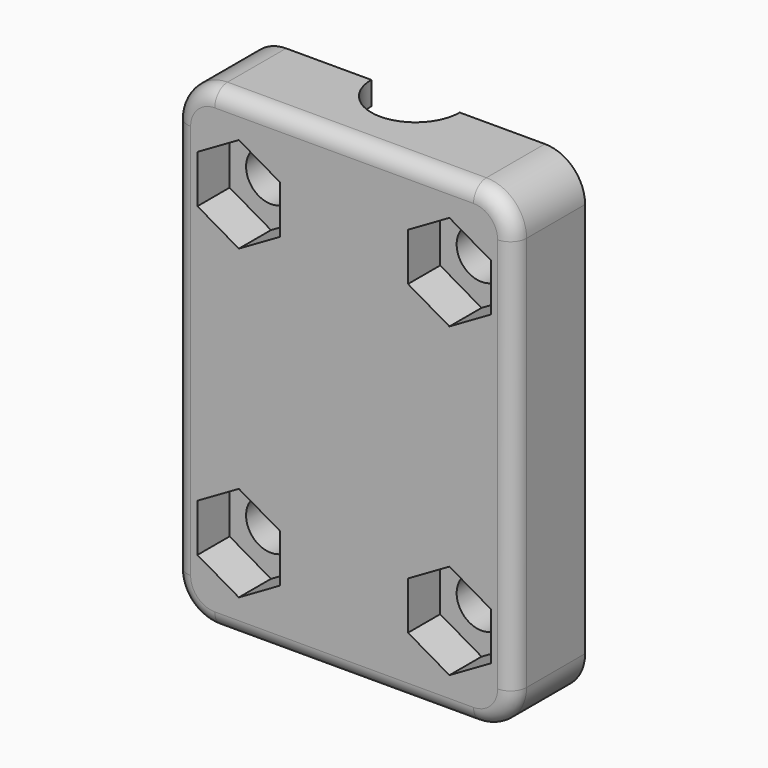
from build123d import *

# Parameters (mm, degrees)
F1_DEPTH = 15.5
F2_DEPTH = 12.6
F3_R     = 3.1
F4_DEPTH = 11.101
F6_R     = 3.1
F7_DEPTH = 5
F9_R     = 5
F10_R    = 2


# Not quite as in the source:
# - a feature names something its author has since deleted; it is built from what else it names


with BuildPart() as f1:
    # F0 (on Top) → F1 (new body, symmetric)
    with BuildSketch(Plane.XY):
        with BuildLine():
            Line((-8.1, 0), (-21.1, 0))
            Line((-21.1, 0), (-21.1, -11.1))
            Line((-21.1, -11.1), (21.1, -11.1))
            Line((21.1, -11.1), (21.1, 0))
            Line((21.1, 0), (8.1, 0))
            ThreePointArc((8.1, 0), (0, -8.1), (-8.1, 0))
        make_face()
        with BuildLine():
            Line((-5.5, 0), (-8.1, 0))
            ThreePointArc((-8.1, 0), (0, -8.1), (8.1, 0))
            Line((8.1, 0), (5.5, 0))
            ThreePointArc((5.5, 0), (0, -5.5), (-5.5, 0))
        make_face()
    extrude(amount=F1_DEPTH, both=True)

    # F0 (on Top) → F2 (cut, symmetric)
    with BuildSketch(Plane.XY):
        with BuildLine():
            Line((-5.5, 0), (-8.1, 0))
            ThreePointArc((-8.1, 0), (0, -8.1), (8.1, 0))
            Line((8.1, 0), (5.5, 0))
            ThreePointArc((5.5, 0), (0, -5.5), (-5.5, 0))
        make_face()
    extrude(amount=F2_DEPTH, both=True, mode=Mode.SUBTRACT)

    # F3 (on Front) → F4 (cut, through all)
    with BuildSketch(Plane.XZ):
        with Locations((13.1, -5)):
            Circle(F3_R)
        with Locations((-13.1, -5)):
            Circle(F3_R)
    extrude(amount=F4_DEPTH, mode=Mode.SUBTRACT)

    # F6 (on face) → F7 (cut)
    with BuildSketch(Plane.XZ.offset(11.1)):
        Polygon((7.95, -2.0266461137), (7.95, -7.9733538863), (13.1, -10.9467077727), (18.25, -7.9733538863), (18.25, -2.0266461137), (13.1, 0.9467077727), align=None)
        with Locations((13.1, -5)):
            Circle(F6_R, mode=Mode.SUBTRACT)
        Polygon((-18.25, -7.9733538863), (-13.1, -10.9467077727), (-7.95, -7.9733538863), (-7.95, -2.0266461137), (-13.1, 0.9467077727), (-18.25, -2.0266461137), align=None)
        with Locations((-13.1, -5)):
            Circle(F6_R, mode=Mode.SUBTRACT)
    extrude(amount=-F7_DEPTH, mode=Mode.SUBTRACT)

    # F8: F1 across plane


with BuildPart() as f1_1:
    add(f1.part)
    add(f1.part.mirror(Plane(origin=(0, -5.9130296111, 14.1), x_dir=(1, 0, 0), z_dir=(0, 0, 1))))

    # F9
    f9_edges = [f1_1.edges().sort_by_distance(p)[0] for p in [
        (21.1, -5.55, 43.7),
        (21.1, -5.55, -15.5),
        (-21.1, -5.55, -15.5),
        (-21.1, -5.55, 43.7),
    ]]
    fillet(f9_edges, radius=F9_R)

    # F10
    f10_edges = [f1_1.edges().sort_by_distance(p)[0] for p in [
        (21.1, -11.1, 14.1),
        (19.635534, -11.1, -14.035534),
        (-21.1, -11.1, 14.1),
        (-19.635534, -11.1, -14.035534),
        (-19.635534, -11.1, 42.235534),
        (0, -11.1, -15.5),
        (0, -11.1, 43.7),
        (19.635534, -11.1, 42.235534),
    ]]
    fillet(f10_edges, radius=F10_R)


solid = f1_1.part
